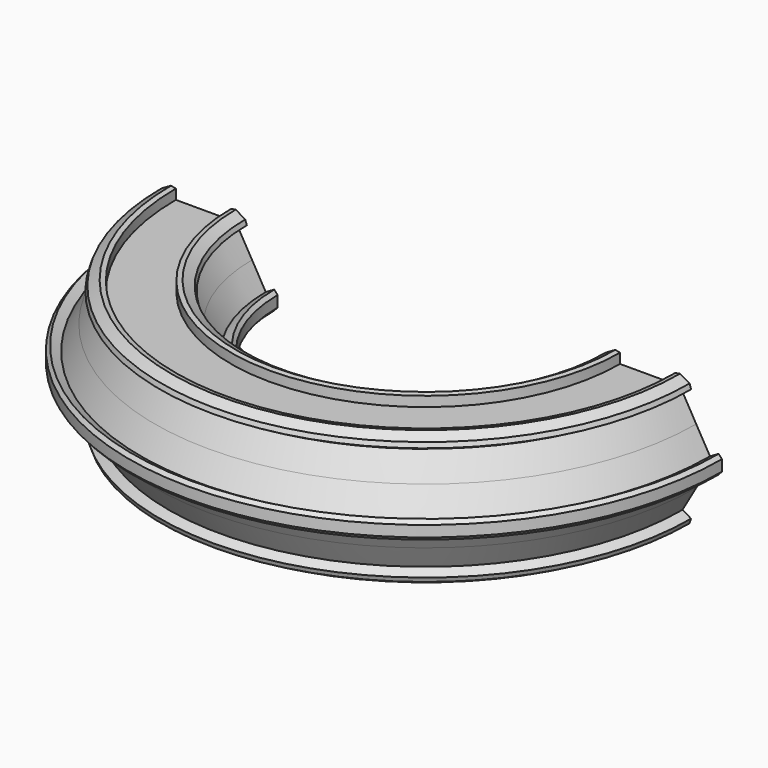
from build123d import *

# Parameters (mm, degrees)
F2_ANGLE = 180


with BuildPart() as f2:
    # F1 (on Front) → F2 (revolve)
    with BuildSketch(Plane.XZ):
        Polygon((-44.861279428, 12.9604106769), (-51.217135042, 12.9604106769), (-57.5630575919, 12.9604106769), (-57.5630575919, 15.2494033683), (-58.6807462598, 15.475716571), (-60.8853201683, 14.20289014), (-61.2508664965, 13.1247800337), (-59.2498548651, 11.9714734282), (-62.425474964, 6.4711380712), (-65.6057968908, 0.9626589096), (-67.5986398816, 2.1112574229), (-68.3491751552, 1.2704479365), (-68.3491751552, -1.2704479365), (-67.590510429, -2.1238883528), (-65.6038210217, -0.9768590888), (-62.4301136979, -6.4738162454), (-59.2582268861, -11.9676853595), (-61.244893976, -13.1146881387), (-60.8774400163, -14.19364456), (-58.6706588228, -15.4396259846), (-57.5584731996, -15.2283469215), (-57.5584731996, -12.9530243576), (-51.217135042, -12.9530243576), (-44.862665236, -12.9530243576), (-44.862665236, -15.2283469215), (-43.7646710275, -15.4396259846), (-41.5434874137, -14.2077057619), (-41.1808964662, -13.1190662144), (-43.1607244284, -11.9802929242), (-39.9959231548, -6.4780897113), (-36.8304619331, -0.9747391376), (-34.850633971, -2.1135124278), (-34.0965986252, -1.2640794445), (-34.1053716838, 1.2640794445), (-34.8630113186, 2.1323707922), (-36.8285001335, 0.9983813071), (-39.9917026714, 6.4810064009), (-43.1661904902, 11.9793805911), (-41.19939244, 13.1149119748), (-41.5604028179, 14.1900196116), (-43.7584016402, 15.4673718757), (-44.861279428, 15.2523063589), align=None)
        Polygon((-60.7503676631, -13.9712226825), (-58.5499524964, -12.7008123937), (-58.5499524964, -15.2283469215), align=None, mode=Mode.SUBTRACT)
        Polygon((-68.0832503253, 1.2704479365), (-65.8827699508, 0), (-68.0832503253, -1.2704479365), align=None, mode=Mode.SUBTRACT)
        Polygon((-43.8843175875, -15.2283469215), (-43.8843175875, -12.7008123937), (-41.6742515512, -13.9767946147), align=None, mode=Mode.SUBTRACT)
        with BuildLine():
            ThreePointArc((-51.217135042, 12.7008123937), (-42.2363044718, 8.9808305702), (-38.5163226482, 0))
            ThreePointArc((-38.5163226482, 0), (-60.1979656121, -8.9808305702), (-51.217135042, 12.7008123937))
        make_face(mode=Mode.SUBTRACT)
        Polygon((-34.3620503103, -1.2640794445), (-36.5515001331, 0), (-34.3620503103, 1.2640794445), align=None, mode=Mode.SUBTRACT)
        Polygon((-58.5499524964, 15.2491778135), (-58.5499524964, 12.7008123937), (-60.7598529608, 13.9766990217), align=None, mode=Mode.SUBTRACT)
        Polygon((-41.6910577545, 13.9670915487), (-43.8843175875, 12.7008123937), (-43.8843175875, 15.2525296435), align=None, mode=Mode.SUBTRACT)
    revolve(axis=Axis((0, 0, 0), (0, 0, 1)), revolution_arc=F2_ANGLE)


solid = f2.part
